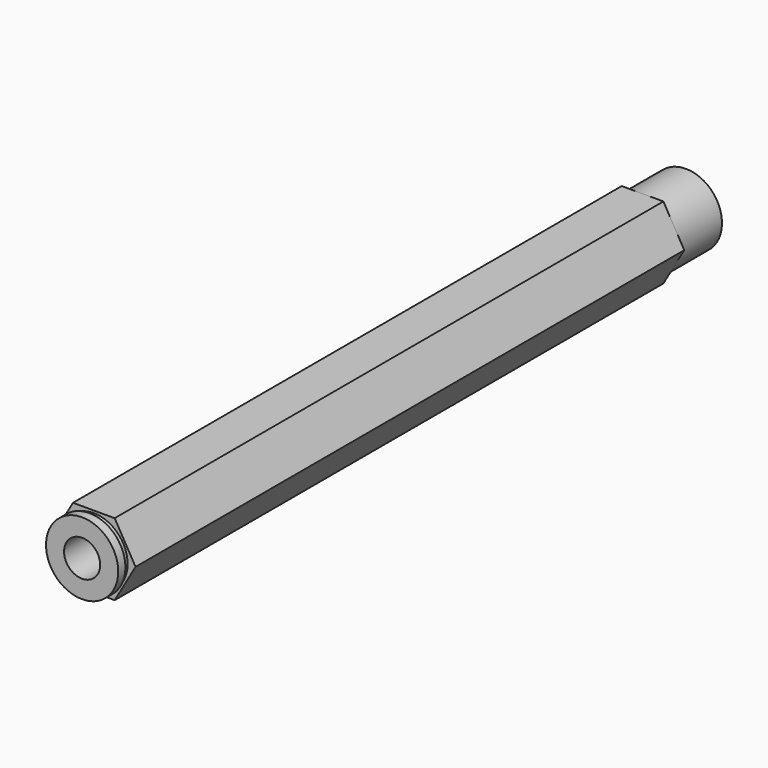
from build123d import *
from build123d import SkipClean  # not in build123d's __all__

# Parameters (mm, degrees)
F1_DEPTH      = 60.325
F1_DEPTH_BACK = 60.325
F2_R          = 5.9436
F3_DEPTH      = 0.9906
F4_R          = 6.35
F5_DEPTH      = 1.5875
F6_R          = 3.175
F7_DEPTH      = 123.2291
F8_R          = 6.35
F8_R_2        = 3.175
F9_DEPTH      = 9.525


with BuildPart() as f1:
    # F0 (on Front) → F1 (new body, two sides)
    with BuildSketch(Plane.XZ) as f1_sk:
        Polygon((3.6661742094, 6.35), (-3.6661742094, 6.35), (-7.3323484187, 0), (-3.6661742094, -6.35), (3.6661742094, -6.35), (7.3323484187, 0), align=None)
    extrude(amount=F1_DEPTH)
    extrude(f1_sk.sketch, amount=-F1_DEPTH_BACK)

    # F2 (on face) → F3 (join)
    with BuildSketch(Plane.XZ.offset(60.325)):
        Circle(F2_R)
    extrude(amount=F3_DEPTH)

    # F4 (on face) → F5 (join)
    with BuildSketch(Plane.XZ.offset(61.3156)):
        Circle(F4_R)
    extrude(amount=F5_DEPTH)

    # F6 (on face) → F7 (cut, through all)
    with BuildSketch(Plane.XZ.offset(62.9031)):
        Circle(F6_R)
    extrude(amount=-F7_DEPTH, mode=Mode.SUBTRACT)

    # F8 (on face) → F9 (join)
    with BuildSketch(Plane(origin=(0, 60.325, 0), x_dir=(-1, 0, 0), z_dir=(0, 1, 0))):
        Circle(F8_R)
        Circle(F8_R_2, mode=Mode.SUBTRACT)
    with SkipClean():  # cleaning this boolean's faces spoils the solid; the shape is the same uncleaned
        extrude(amount=F9_DEPTH)


solid = f1.part
